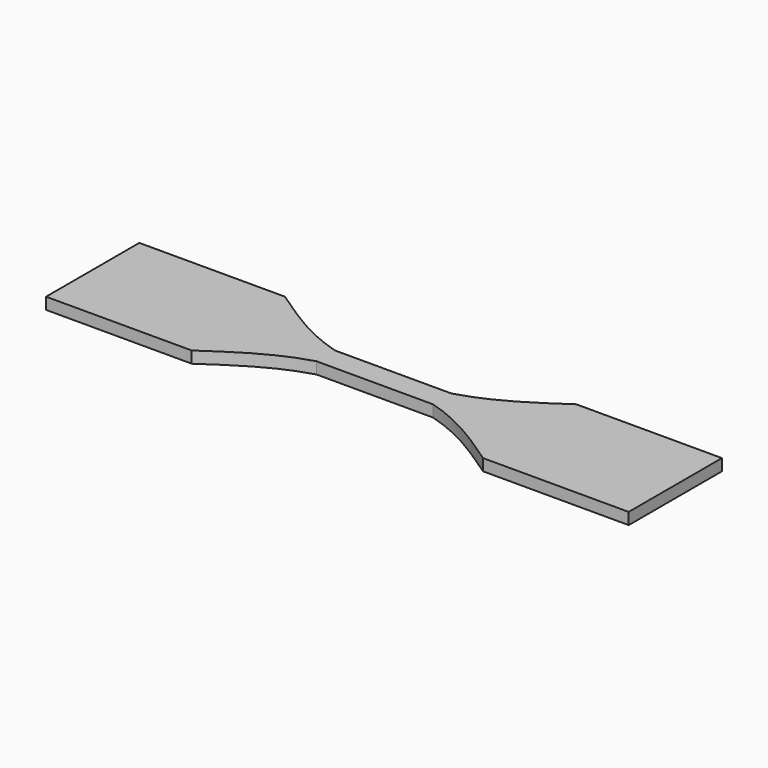
from build123d import *

# Parameters (mm, degrees)
F1_DEPTH = 1


with BuildPart() as f1:
    # F0 (on Top) → F1 (new body)
    with BuildSketch(Plane.XY):
        with BuildLine():
            Line((-12.5, 5), (-20, 5))
            Line((-20, 5), (-25, 5))
            Line((-25, 5), (-25, -5))
            Line((-25, -5), (-20, -5))
            Line((-20, -5), (-12.5, -5))
            add(Edge.make_bspline(
                [(-5, -1), (-7.8716344223, -1.8257793632), (-10.1858172112, -3.4128896816), (-12.5, -5)],
                knots=[0.6758143524, 0.6758143524, 0.6758143524, 0.6758143524, 1, 1, 1, 1], degree=3))
            add(Edge.make_bspline(
                [(5, -1), (1.8852751504, -0.1043165234), (-1.8852751504, -0.1043165234), (-5, -1)],
                knots=[0.3241856476, 0.3241856476, 0.3241856476, 0.3241856476, 0.6758143524, 0.6758143524, 0.6758143524, 0.6758143524], degree=3))
            add(Edge.make_bspline(
                [(12.5, -5), (10.1858172112, -3.4128896816), (7.8716344223, -1.8257793632), (5, -1)],
                knots=[0, 0, 0, 0, 0.3241856476, 0.3241856476, 0.3241856476, 0.3241856476], degree=3))
            Line((12.5, -5), (20, -5))
            Line((20, -5), (25, -5))
            Line((25, -5), (25, 5))
            Line((25, 5), (20, 5))
            Line((20, 5), (12.5, 5))
            add(Edge.make_bspline(
                [(5, 1), (7.8716344223, 1.8257793632), (10.1858172112, 3.4128896816), (12.5, 5)],
                knots=[0.6758143524, 0.6758143524, 0.6758143524, 0.6758143524, 1, 1, 1, 1], degree=3))
            add(Edge.make_bspline(
                [(-5, 1), (-1.8852751504, 0.1043165234), (1.8852751504, 0.1043165234), (5, 1)],
                knots=[0.3241856476, 0.3241856476, 0.3241856476, 0.3241856476, 0.6758143524, 0.6758143524, 0.6758143524, 0.6758143524], degree=3))
            add(Edge.make_bspline(
                [(-12.5, 5), (-10.1858172112, 3.4128896816), (-7.8716344223, 1.8257793632), (-5, 1)],
                knots=[0, 0, 0, 0, 0.3241856476, 0.3241856476, 0.3241856476, 0.3241856476], degree=3))
        make_face()
        with BuildLine():
            Line((5, 1), (-5, 1))
            add(Edge.make_bspline(
                [(-5, 1), (-1.8852751504, 0.1043165234), (1.8852751504, 0.1043165234), (5, 1)],
                knots=[0.3241856476, 0.3241856476, 0.3241856476, 0.3241856476, 0.6758143524, 0.6758143524, 0.6758143524, 0.6758143524], degree=3))
        make_face()
        with BuildLine():
            add(Edge.make_bspline(
                [(5, -1), (1.8852751504, -0.1043165234), (-1.8852751504, -0.1043165234), (-5, -1)],
                knots=[0.3241856476, 0.3241856476, 0.3241856476, 0.3241856476, 0.6758143524, 0.6758143524, 0.6758143524, 0.6758143524], degree=3))
            Line((-5, -1), (5, -1))
        make_face()
    extrude(amount=F1_DEPTH)


solid = f1.part
